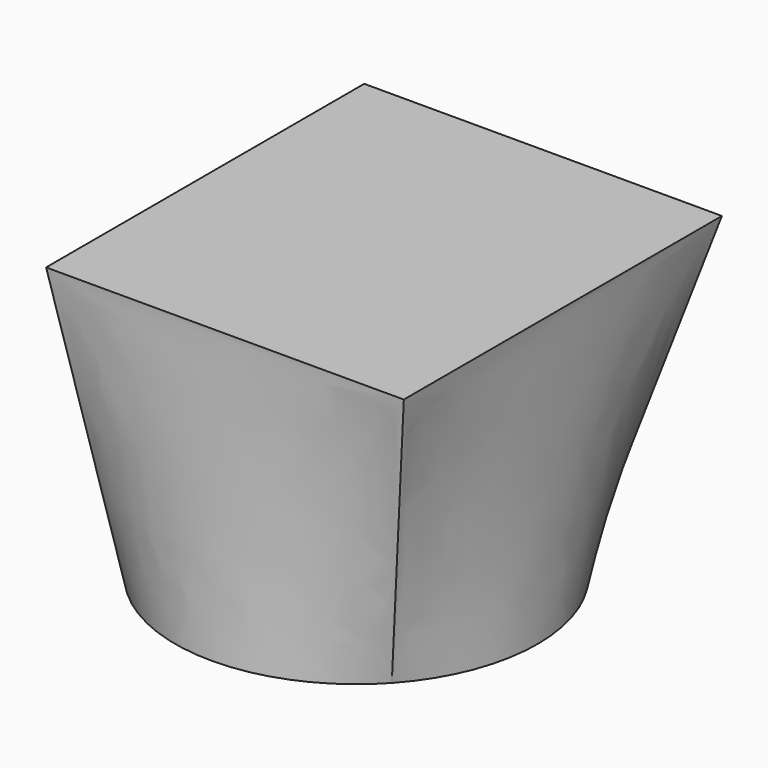
from build123d import *

# Parameters (mm, degrees)
F2_W = 65.2415901423
F2_H = 72.5182639435


# Not quite as in the source:
# - the arcs of a loft's sections are written as splines that run evenly, so that the points pair up as in the source's solid


with BuildPart() as f3:
    # F1 (on Top) → F3 section 0
    with BuildSketch(Plane.XY):
        with BuildLine():
            add(Edge.make_bspline(
                [(24.3328670737, -22.365063842), (25.7966570792, -20.7724814162), (27.1035590901, -19.0357712032), (29.3534916354, -15.3406658739), (30.2964665359, -13.3823621265), (31.7822879698, -9.3193171453), (32.3250977633, -7.2146763783), (32.9897088011, -2.9398322851), (33.1114936117, -0.7697346629), (32.9293536241, 3.5526286812), (32.6254333297, 5.704787524), (31.6035418543, 9.9085641195), (30.8855959415, 11.9600779256), (29.0632236945, 15.8837189956), (27.9588424221, 17.7557492398), (25.406022147, 21.2484714583), (23.9576462679, 22.8690770682), (22.365063842, 24.3328670737)],
                knots=[0, 0, 0, 0, 0.125, 0.125, 0.25, 0.25, 0.375, 0.375, 0.5, 0.5, 0.625, 0.625, 0.75, 0.75, 0.875, 0.875, 1, 1, 1, 1], degree=3))
            add(Edge.make_bspline(
                [(22.365063842, 24.3328670737), (20.7724814162, 25.7966570792), (19.0357712032, 27.1035590901), (15.3406658739, 29.3534916354), (13.3823621265, 30.2964665359), (9.3193171453, 31.7822879698), (7.2146763783, 32.3250977633), (2.9398322851, 32.9897088011), (0.7697346629, 33.1114936117), (-3.5526286812, 32.9293536241), (-5.704787524, 32.6254333297), (-9.9085641195, 31.6035418543), (-11.9600779256, 30.8855959415), (-15.8837189956, 29.0632236945), (-17.7557492398, 27.9588424221), (-21.2484714583, 25.406022147), (-22.8690770682, 23.9576462679), (-24.3328670737, 22.365063842)],
                knots=[0, 0, 0, 0, 0.125, 0.125, 0.25, 0.25, 0.375, 0.375, 0.5, 0.5, 0.625, 0.625, 0.75, 0.75, 0.875, 0.875, 1, 1, 1, 1], degree=3))
            add(Edge.make_bspline(
                [(-24.3328670737, 22.365063842), (-25.7966570792, 20.7724814162), (-27.1035590901, 19.0357712032), (-29.3534916354, 15.3406658739), (-30.2964665359, 13.3823621265), (-31.7822879698, 9.3193171453), (-32.3250977633, 7.2146763783), (-32.9897088011, 2.9398322851), (-33.1114936117, 0.7697346629), (-32.9293536241, -3.5526286812), (-32.6254333297, -5.704787524), (-31.6035418543, -9.9085641195), (-30.8855959415, -11.9600779256), (-29.0632236945, -15.8837189956), (-27.9588424221, -17.7557492398), (-25.406022147, -21.2484714583), (-23.9576462679, -22.8690770682), (-22.365063842, -24.3328670737)],
                knots=[0, 0, 0, 0, 0.125, 0.125, 0.25, 0.25, 0.375, 0.375, 0.5, 0.5, 0.625, 0.625, 0.75, 0.75, 0.875, 0.875, 1, 1, 1, 1], degree=3))
            add(Edge.make_bspline(
                [(-22.365063842, -24.3328670737), (-20.7724814162, -25.7966570792), (-19.0357712032, -27.1035590901), (-15.3406658739, -29.3534916354), (-13.3823621265, -30.2964665359), (-9.3193171453, -31.7822879698), (-7.2146763783, -32.3250977633), (-2.9398322851, -32.9897088011), (-0.7697346629, -33.1114936117), (3.5526286812, -32.9293536241), (5.704787524, -32.6254333297), (9.9085641195, -31.6035418543), (11.9600779256, -30.8855959415), (15.8837189956, -29.0632236945), (17.7557492398, -27.9588424221), (21.2484714583, -25.406022147), (22.8690770682, -23.9576462679), (24.3328670737, -22.365063842)],
                knots=[0, 0, 0, 0, 0.125, 0.125, 0.25, 0.25, 0.375, 0.375, 0.5, 0.5, 0.625, 0.625, 0.75, 0.75, 0.875, 0.875, 1, 1, 1, 1], degree=3))
        make_face()
    # F2 (on offset) → F3 section 1
    with BuildSketch(Plane.XY.offset(51.3)):
        with Locations((0, 6.2763863243)):
            Rectangle(F2_W, F2_H)
    loft(ruled=True)


solid = f3.part
